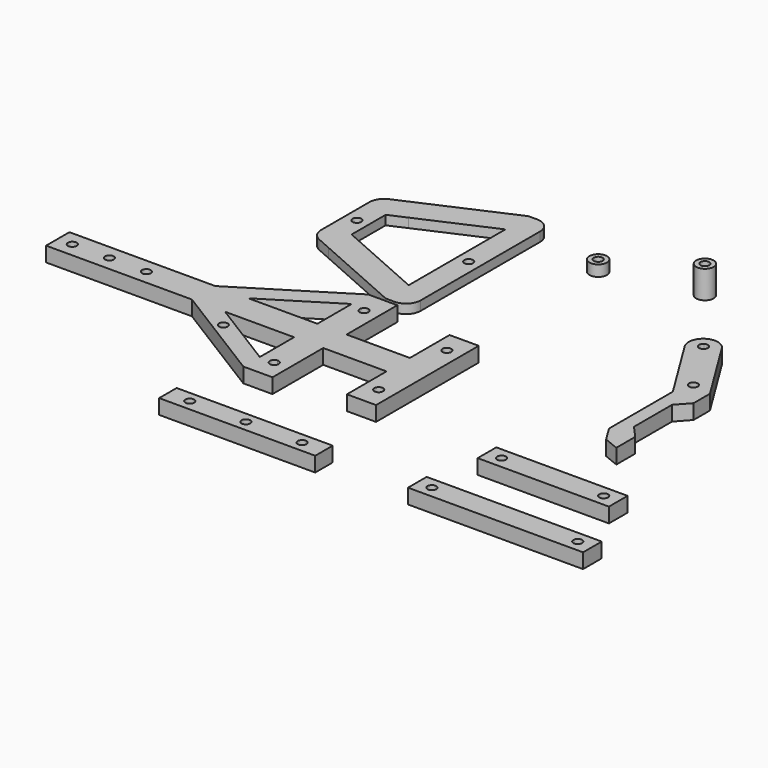
from build123d import *

# Parameters (mm, degrees)
F0_W     = 8
F0_H     = 19.684662618
F0_R     = 1.5
F0_H_2   = 10.8739659115
F1_DEPTH = 3.18
F0_R_2   = 3
F2_DEPTH = 3.762
F3_DEPTH = 5.08
F0_W_2   = 53.5
F0_H_3   = 7.5
F0_W_3   = 5
F0_H_4   = 5
F0_W_4   = 16.7056103051
F0_H_5   = 10
F0_W_5   = 22.5
F0_H_6   = 8
F0_W_6   = 30
F4_R     = 4.99999
F5_DEPTH = 9.525
F6_R     = 5


# Not quite as in the source:
# - a fillet or chamfer is up to 0.001 mm smaller than in the source, because OpenCascade refuses the exact size
# - a feature names something its author has since deleted; it is built from what else it names


with BuildPart() as f1:
    # F0 (on Top) → F1 (new body)
    with BuildSketch(Plane.XY):
        with Locations((-57.7275006586, 75.0977412903)):
            Rectangle(F0_W, F0_H)
        with Locations((-57.7275006586, 75.0977412903)):
            Circle(F0_R, mode=Mode.SUBTRACT)
        with Locations((-57.7275006586, 90.3770555551)):
            Rectangle(F0_W, F0_H_2)
        Polygon((-61.7275006586, 95.8140385108), (-53.7275006586, 95.8140385108), (-53.7275006586, 105.6563698198), (-61.7275006586, 105.6563698198), (-92.0275006586, 92.2438953373), (-92.0275006586, 84.9400725994), (-86.2927788664, 84.9400725994), align=None)
        with Locations((-57.7275006586, 59.8184270256)):
            Rectangle(F0_W, F0_H_2)
        Polygon((-92.0275006586, 82.4015640283), (-86.2927788664, 84.9400725994), (-92.0275006586, 84.9400725994), align=None)
        Polygon((-53.7275006586, 44.5391127608), (-53.7275006586, 54.3814440698), (-61.7275006586, 54.3814440698), (-86.2927788664, 65.2554099813), (-92.0275006586, 65.2554099813), (-92.0275006586, 57.9515872433), (-61.7275006586, 44.5391127608), align=None)
        Polygon((-92.0275006586, 82.4015640283), (-92.0275006586, 84.9400725994), (-100.0275006586, 84.9400725994), (-100.0275006586, 78.8603166402), align=None)
        Polygon((-100.0275006586, 84.9400725994), (-92.0275006586, 84.9400725994), (-92.0275006586, 92.2438953373), (-100.0275006586, 88.7026479492), align=None)
        Polygon((-92.0275006586, 67.7939185523), (-92.0275006586, 82.4015640283), (-100.0275006586, 78.8603166402), (-100.0275006586, 71.3351659405), align=None)
        with Locations((-96.0275006586, 75.0977412903)):
            Circle(F0_R, mode=Mode.SUBTRACT)
        Polygon((-92.0275006586, 65.2554099813), (-86.2927788664, 65.2554099813), (-92.0275006586, 67.7939185523), align=None)
        Polygon((-92.0275006586, 65.2554099813), (-92.0275006586, 67.7939185523), (-100.0275006586, 71.3351659405), (-100.0275006586, 65.2554099813), align=None)
        Polygon((-92.0275006586, 57.9515872433), (-92.0275006586, 65.2554099813), (-100.0275006586, 65.2554099813), (-100.0275006586, 61.4928346314), align=None)
    extrude(amount=F1_DEPTH)

    # F6
    f6_edges = [f1.edges().sort_by_distance(p)[0] for p in [
        (-100.027501, 61.492835, 1.59),
        (-100.027501, 88.702648, 1.59),
        (-53.727501, 105.65637, 1.59),
        (-53.727501, 44.539113, 1.59),
    ]]
    fillet(f6_edges, radius=F6_R)


with BuildPart() as f2:
    # F0 (on Top) → F2 (new body)
    with BuildSketch(Plane.XY):
        with Locations((-30.7930689305, 96.9169214368)):
            Circle(F0_R_2)
        with Locations((-30.7930689305, 96.9169214368)):
            Circle(F0_R, mode=Mode.SUBTRACT)
    extrude(amount=F2_DEPTH)


with BuildPart() as f3:
    # F0 (on Top) → F3 (new body)
    with BuildSketch(Plane.XY):
        with BuildLine():
            ThreePointArc((23.5557945233, 74.3777250811), (25.0755266494, 74.4131629436), (25.8458071751, 73.1026250811))
            ThreePointArc((25.8458071751, 73.1026250811), (24.756507796, 71.659945283), (23.0707071751, 72.3126124293))
            Line((23.0707071751, 72.3126124293), (20.0954738417, 70.4692495751))
            Line((20.0954738417, 70.4692495751), (26.0205687302, 60.9059995751))
            Line((26.0205687302, 60.9059995751), (31.9456636187, 51.3427495751))
            Line((31.9456636187, 51.3427495751), (34.3157015741, 47.5174495751))
            Line((34.3157015741, 47.5174495751), (38.5660349074, 50.1508250811))
            Line((38.5660349074, 50.1508250811), (42.8163682408, 52.7842005871))
            Line((42.8163682408, 52.7842005871), (40.4463302854, 56.6095005871))
            Line((40.4463302854, 56.6095005871), (28.5961405084, 75.7360005871))
            Line((28.5961405084, 75.7360005871), (26.226102553, 79.5613005871))
            Line((26.226102553, 79.5613005871), (21.9757692197, 76.9279250811))
            Line((21.9757692197, 76.9279250811), (23.5557945233, 74.3777250811))
        make_face()
        with Locations((36.195996952, 53.9761250811)):
            Circle(F0_R, mode=Mode.SUBTRACT)
        with BuildLine():
            ThreePointArc((23.0707071751, 72.3126124293), (22.8855520151, 73.4456336345), (23.5557945233, 74.3777250811))
            Line((23.5557945233, 74.3777250811), (21.9757692197, 76.9279250811))
            Line((21.9757692197, 76.9279250811), (17.7254358863, 74.2945495751))
            Line((17.7254358863, 74.2945495751), (20.0954738417, 70.4692495751))
            Line((20.0954738417, 70.4692495751), (23.0707071751, 72.3126124293))
        make_face()
        Polygon((38.5660349074, 50.1508250811), (34.3157015741, 47.5174495751), (34.3157015741, 33.2842005871), (38.8978719711, 33.2842005871), (38.8978719711, 41.4348132908), (38.8978719711, 45.7842005871), (42.8163682408, 45.7842005871), (42.8163682408, 52.7842005871), align=None)
        Polygon((38.8978719711, 41.4348132908), (42.8163682408, 45.7842005871), (38.8978719711, 45.7842005871), align=None)
        Polygon((38.8978719711, 33.2842005871), (34.3157015741, 33.2842005871), (34.3157015741, 20.1585646719), (37.6538338433, 14.7707364557), (42.8163682408, 12.6621089876), (42.8163682408, 20.7842005871), (38.8978719711, 20.7842005871), (38.8978719711, 25.1335878834), align=None)
        Polygon((42.8163682408, 20.7842005871), (38.8978719711, 25.1335878834), (38.8978719711, 20.7842005871), align=None)
    extrude(amount=F3_DEPTH)

    # F4 (radius 5 in the source; OpenCascade refuses exactly that, so slightly less here)
    f4_edges = [f3.edges().sort_by_distance(p)[0] for p in [
        (17.725436, 74.29455, 2.54),
        (26.226103, 79.561301, 2.54),
    ]]
    fillet(f4_edges, radius=F4_R)


with BuildPart() as f3b:
    # F0 (on Top) → F3, piece 2 (new body)
    with BuildSketch(Plane.XY):
        with Locations((-43.9775006586, -37.5333949924)):
            Rectangle(F0_W_2, F0_H_3)
        with Locations((-63.2275006586, -37.5333949924)):
            Circle(F0_R, mode=Mode.SUBTRACT)
        with BuildLine():
            ThreePointArc((-42.4775006586, -37.5333949924), (-43.9775006586, -39.0333949924), (-45.4775006586, -37.5333949924))
            ThreePointArc((-45.4775006586, -37.5333949924), (-43.9775006586, -36.0333949924), (-42.4775006586, -37.5333949924))
        make_face(mode=Mode.SUBTRACT)
        with BuildLine():
            ThreePointArc((-23.2275006586, -37.5333949924), (-24.7275006586, -39.0333949924), (-26.2275006586, -37.5333949924))
            ThreePointArc((-26.2275006586, -37.5333949924), (-24.7275006586, -36.0333949924), (-23.2275006586, -37.5333949924))
        make_face(mode=Mode.SUBTRACT)
    extrude(amount=F3_DEPTH)


with BuildPart() as f3c:
    # F0 (on Top) → F3, piece 3 (new body)
    with BuildSketch(Plane.XY):
        Polygon((-99.5664379767, 18.8185117334), (-88.1988368955, 18.8185117334), (-64.5664379767, 33.504359633), (-64.5664379767, 40.5685117334), align=None)
        Polygon((-64.5664379767, 33.504359633), (-64.5664379767, 18.8185117334), (-59.5664379767, 18.8185117334), (-54.5664379767, 18.8185117334), (-54.5664379767, 40.5685117334), (-64.5664379767, 40.5685117334), align=None)
        with BuildLine():
            ThreePointArc((-58.0664379767, 32.5685117334), (-58.5057778049, 31.5078515616), (-59.5664379767, 31.0685117334))
            ThreePointArc((-59.5664379767, 31.0685117334), (-60.6270981485, 33.6291719052), (-58.0664379767, 32.5685117334))
        make_face(mode=Mode.SUBTRACT)
        with Locations((-62.0664379767, 16.3185117334)):
            Rectangle(F0_W_3, F0_H_4)
        with Locations((-57.0664379767, 16.3185117334)):
            Rectangle(F0_W_3, F0_H_4)
        Polygon((-59.5664379767, 8.8185117334), (-64.5664379767, 8.8185117334), (-64.5664379767, -5.8673361662), (-64.5664379767, -12.9314882666), (-54.5664379767, -12.9314882666), (-54.5664379767, 8.8185117334), align=None)
        with BuildLine():
            ThreePointArc((-58.0664379767, -5.9314882666), (-60.6270981485, -6.9921484384), (-59.5664379767, -4.4314882666))
            ThreePointArc((-59.5664379767, -4.4314882666), (-58.5057778049, -4.8708280948), (-58.0664379767, -5.9314882666))
        make_face(mode=Mode.SUBTRACT)
        Polygon((-64.5664379767, 18.8185117334), (-88.1988368955, 18.8185117334), (-99.5664379767, 18.8185117334), (-149.5664379767, 18.8185117334), (-149.5664379767, 8.8185117334), (-99.5664379767, 8.8185117334), (-88.1988368955, 8.8185117334), (-64.5664379767, 8.8185117334), (-64.5664379767, 13.8185117334), align=None)
        with Locations((-144.5664379767, 13.8185117334)):
            Circle(F0_R, mode=Mode.SUBTRACT)
        with Locations((-131.8664379767, 13.8185117334)):
            Circle(F0_R, mode=Mode.SUBTRACT)
        with Locations((-119.1664379767, 13.8185117334)):
            Circle(F0_R, mode=Mode.SUBTRACT)
        with Locations((-57.0664379767, 11.3185117334)):
            Rectangle(F0_W_3, F0_H_4)
        with Locations((-62.0664379767, 11.3185117334)):
            Rectangle(F0_W_3, F0_H_4)
        Polygon((-49.5664379767, 18.8185117334), (-54.5664379767, 18.8185117334), (-54.5664379767, 13.8185117334), (-54.5664379767, 8.8185117334), (-49.5664379767, 8.8185117334), align=None)
        with Locations((-41.2136328242, 13.8185117334)):
            Rectangle(F0_W_4, F0_H_5)
        Polygon((-32.8608276716, 35.822091948), (-32.8608276716, 18.8185117334), (-27.8608276716, 18.8185117334), (-27.8608276716, 8.8185117334), (-32.8608276716, 8.8185117334), (-32.8608276716, -8.1850684811), (-22.8608276716, -8.1850684811), (-22.8608276716, 35.822091948), align=None)
        with Locations((-27.8608276716, -0.7780961324)):
            Circle(F0_R, mode=Mode.SUBTRACT)
        with Locations((-27.8608276716, 28.4151195993)):
            Circle(F0_R, mode=Mode.SUBTRACT)
        with Locations((-30.3608276716, 13.8185117334)):
            Rectangle(F0_W_3, F0_H_5)
        with BuildLine():
            Line((-88.1988368955, 8.8185117334), (-99.5664379767, 8.8185117334))
            Line((-99.5664379767, 8.8185117334), (-85.3757294402, 0))
            Line((-85.3757294402, 0), (-84.5840056687, 1.2740382529))
            ThreePointArc((-84.5840056687, 1.2740382529), (-85.0663201502, 3.3398002772), (-83.0005581259, 3.8221147586))
            Line((-83.0005581259, 3.8221147586), (-82.2088343545, 5.0961530115))
            Line((-82.2088343545, 5.0961530115), (-88.1988368955, 8.8185117334))
        make_face()
        with BuildLine():
            Line((-64.5664379767, -12.9314882666), (-64.5664379767, -5.8673361662))
            Line((-64.5664379767, -5.8673361662), (-82.2088343545, 5.0961530115))
            Line((-82.2088343545, 5.0961530115), (-83.0005581259, 3.8221147586))
            ThreePointArc((-83.0005581259, 3.8221147586), (-82.481254503, 3.2769161118), (-82.2922818973, 2.5480765057))
            ThreePointArc((-82.2922818973, 2.5480765057), (-83.0634422912, 1.2370491114), (-84.5840056687, 1.2740382529))
            Line((-84.5840056687, 1.2740382529), (-85.3757294402, 0))
            Line((-85.3757294402, 0), (-64.5664379767, -12.9314882666))
        make_face()
    extrude(amount=F3_DEPTH)


with BuildPart() as f3d:
    # F0 (on Top) → F3, piece 4 (new body)
    with BuildSketch(Plane.XY):
        with Locations((28.8328784704, -11.2028054856)):
            Rectangle(F0_W_5, F0_H_6)
        with Locations((22.5828784704, -11.2028054856)):
            Circle(F0_R, mode=Mode.SUBTRACT)
        with Locations((51.3328784704, -11.2028054856)):
            Rectangle(F0_W_5, F0_H_6)
        with Locations((57.5828784704, -11.2028054856)):
            Circle(F0_R, mode=Mode.SUBTRACT)
    extrude(amount=F3_DEPTH)


with BuildPart() as f3e:
    # F0 (on Top) → F3, piece 5 (new body)
    with BuildSketch(Plane.XY):
        with Locations((58.7242078781, -36.2158461511)):
            Rectangle(F0_W_6, F0_H_6)
        with Locations((68.7242078781, -36.2158461511)):
            Circle(F0_R, mode=Mode.SUBTRACT)
        with Locations((28.7242078781, -36.2158461511)):
            Rectangle(F0_W_6, F0_H_6)
        with Locations((18.7242078781, -36.2158461511)):
            Circle(F0_R, mode=Mode.SUBTRACT)
    extrude(amount=F3_DEPTH)


with BuildPart() as f5:
    # F0 (on Top) → F5 (new body)
    with BuildSketch(Plane.XY):
        with Locations((0, 104.1563698198)):
            Circle(F0_R_2)
        with Locations((0, 104.1563698198)):
            Circle(F0_R, mode=Mode.SUBTRACT)
    extrude(amount=F5_DEPTH)


solid = Compound([f1.part, f2.part, f3.part, f3b.part, f3c.part, f3d.part, f3e.part, f5.part])
